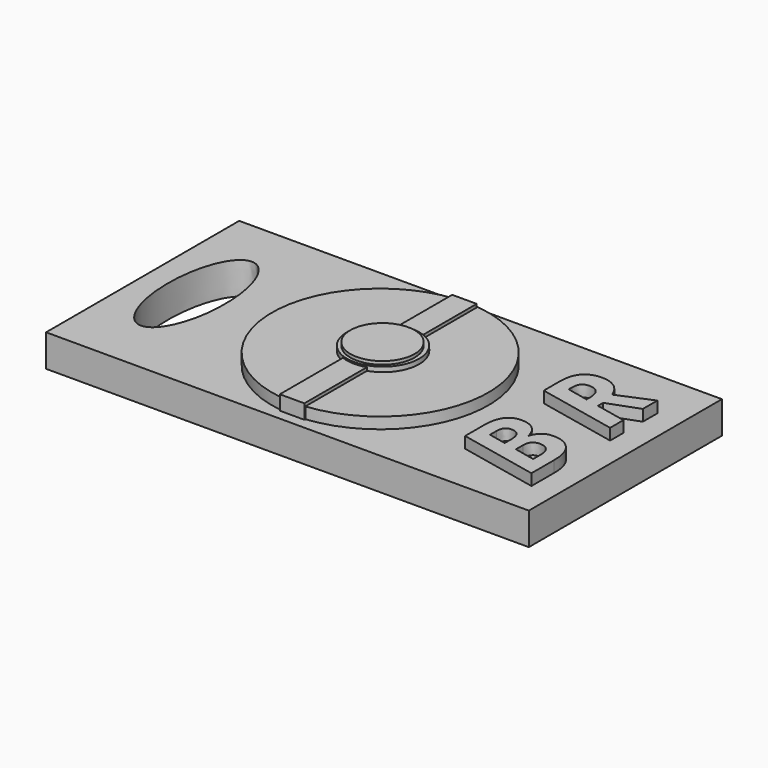
from build123d import *

# Parameters (mm, degrees)
F0_W          = 76.2
F0_H          = 38.1
F1_DEPTH      = 5.08
F3_DEPTH      = 25.4
F4_R          = 17.0880639947
F5_DEPTH      = 6.858
F6_W          = 3.8722375175
F6_H          = 34.0030835941
F7_DEPTH      = 7.366
F8_R          = 5.6944727458
F9_DEPTH      = 7.62
F10_R         = 5.0774489709
F11_DEPTH     = 8.128
F12_TEXT_SIZE = 17.6388888889
F13_DEPTH     = 6.858


# Not quite as in the source:
# - Text() gives the source's letters only with a copy of the font that has no kerning and outlines rounded to 1/6400 em; it was checked with that copy


with BuildPart() as f1:
    # F0 (on Top) → F1 (new body)
    with BuildSketch(Plane.XY):
        with Locations((0.4317108542, 3.4453301371)):
            Rectangle(F0_W, F0_H)
    extrude(amount=F1_DEPTH)

    # F2 (on Top) → F3 (cut)
    with BuildSketch(Plane.XY):
        with BuildLine():
            add(Edge.make_bspline(
                [(-29.6439919621, -6.9054194939), (-21.8866543054, -6.9054194939), (-25.7653231338, 9.4966305061), (-29.6439919621, 25.8986805061), (-33.5226607904, 9.4966305061), (-37.4013296187, -6.9054194939), (-29.6439919621, -6.9054194939)],
                knots=[0, 0, 0, 2.0943951024, 2.0943951024, 4.1887902048, 4.1887902048, 6.2831853072, 6.2831853072, 6.2831853072], degree=2, weights=[1, 0.5, 1, 0.5, 1, 0.5, 1]))
        make_face()
    extrude(amount=F3_DEPTH, mode=Mode.SUBTRACT)

    # F4 (on Top) → F5 (join)
    with BuildSketch(Plane.XY):
        with Locations((0, 3.2269193325)):
            Circle(F4_R)
    extrude(amount=F5_DEPTH)

    # F6 (on Top) → F7 (join)
    with BuildSketch(Plane.XY):
        with Locations((-0.1548785367, 3.0471025966)):
            Rectangle(F6_W, F6_H)
    extrude(amount=F7_DEPTH)

    # F8 (on Top) → F9 (join)
    with BuildSketch(Plane.XY):
        with Locations((0, 3.8022240624)):
            Circle(F8_R)
    extrude(amount=F9_DEPTH)

    # F10 (on Top) → F11 (join)
    with BuildSketch(Plane.XY):
        with Locations((0, 3.689033445)):
            Circle(F10_R)
    extrude(amount=F11_DEPTH)

    # F12 (on Top) → F13 (join)
    with BuildSketch(Plane.XY):
        with Locations(Location((34.6810782016, -10.7355244217), (0, 0, 90))):
            Text('B R', F12_TEXT_SIZE, font='Open Sans', font_style=FontStyle.BOLDITALIC, text_align=(TextAlign.LEFT, TextAlign.BOTTOM))
    extrude(amount=F13_DEPTH)


solid = f1.part
